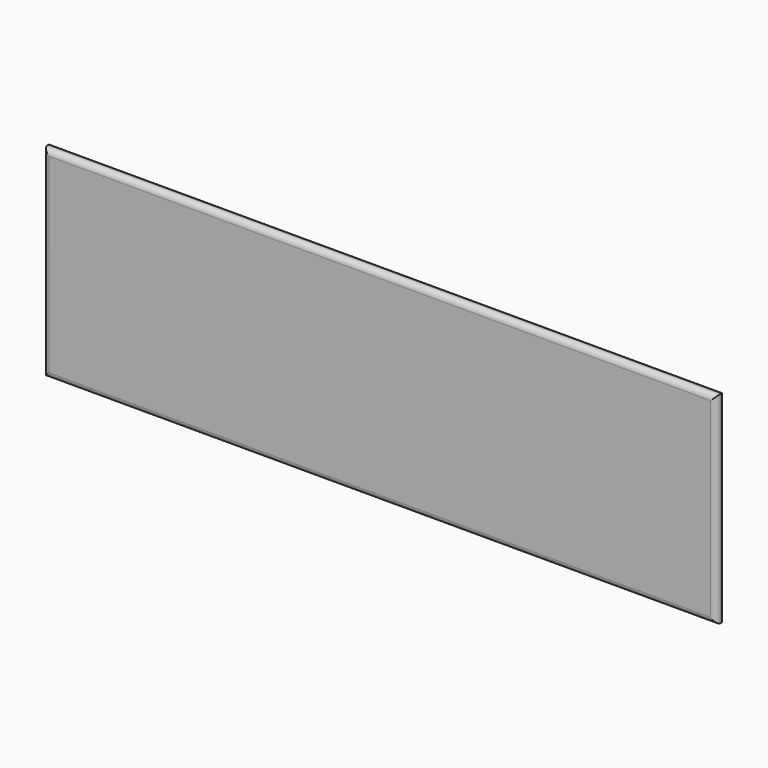
from build123d import *

# Parameters (mm, degrees)
F0_W     = 1524
F0_H     = 457.2
F1_DEPTH = 15.875
F2_R     = 12.7
F4_D     = 12.7
F4_DEPTH = 9.525
F4_TIP   = 3.8154649308


# Not quite as in the source:
# - a length typed as a fraction of an inch, garbled in the dataset ("3 / 203.2 mm" for 3/8 in), is restored


with BuildPart() as f1:
    # F0 (on Front) → F1 (new body)
    with BuildSketch(Plane.XZ):
        Rectangle(F0_W, F0_H)
    extrude(amount=F1_DEPTH)

    # F2
    f2_edges = [f1.edges().sort_by_distance(p)[0] for p in [
        (0, -15.875, 228.6),
        (-762, -15.875, 0),
        (0, -15.875, -228.6),
        (762, -15.875, 0),
    ]]
    fillet(f2_edges, radius=F2_R)

    # F4
    with Locations(Plane(origin=(0, 0, 0), x_dir=(-1, 0, 0), z_dir=(0, 1, 0))):
        with Locations((-711.2, 177.8), (-711.2, -186.6344660521), (711.2, -186.6344660521), (711.2, 177.8)):
            Hole(F4_D / 2, depth=F4_DEPTH)
            with Locations((0, 0, -(F4_DEPTH + F4_TIP / 2))):  # 118° drill point
                Cone(0, F4_D / 2, F4_TIP, mode=Mode.SUBTRACT)


solid = f1.part
